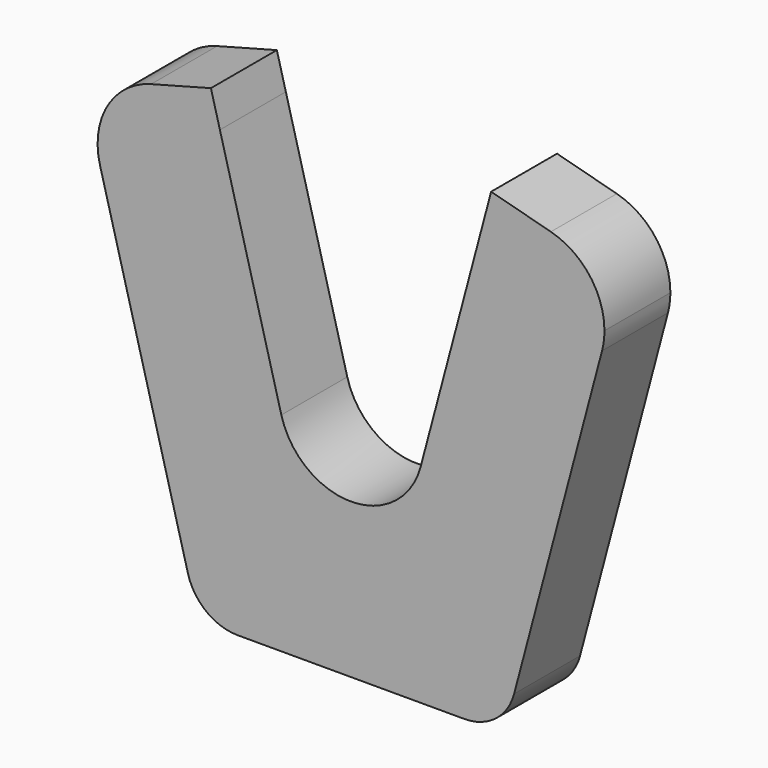
from build123d import *

# Parameters (mm, degrees)
F1_DEPTH = 25.4


with BuildPart() as f1:
    # F0 (on Front) → F1 (new body)
    with BuildSketch(Plane.XZ):
        with BuildLine():
            ThreePointArc((-96.2938510095, 49.8640834202), (-106.1566639379, 55.4102805892), (-117.4718999148, 55.3817029315))
            ThreePointArc((-117.4718999148, 55.3817029315), (-130.9864974324, 45.0518805264), (-133.238473511, 28.1913295056))
            ThreePointArc((-133.238473511, 28.1913295056), (-111.9975569081, 11.6794990469), (-90.4085331471, 27.7335059074))
            Line((-90.4085331471, 27.7335059074), (-96.2938510095, 49.8640834202))
        make_face()
        with BuildLine():
            Line((-99.0630919931, 60.2772681748), (-117.4718999148, 55.3817029315))
            ThreePointArc((-117.4718999148, 55.3817029315), (-106.1566639379, 55.4102805892), (-96.2938510095, 49.8640834202))
            Line((-96.2938510095, 49.8640834202), (-99.0630919931, 60.2772681748))
        make_face()
        with BuildLine():
            ThreePointArc((-90.4085331471, 27.7335059074), (-111.9975569081, 11.6794990469), (-133.238473511, 28.1913295056))
            Line((-133.238473511, 28.1913295056), (-106.1467650121, -73.6816990901))
            ThreePointArc((-106.1467650121, -73.6816990901), (-92.8623116551, -53.860643351), (-74.9299982186, -69.6017705795))
            ThreePointArc((-74.9299982186, -69.6017705795), (-79.5796780672, -80.8270907309), (-90.8049982186, -85.4767705795))
            Line((-90.8049982186, -85.4767705795), (-20.9549982186, -85.4767705795))
            ThreePointArc((-20.9549982186, -85.4767705795), (-32.1803231924, -58.3764516879), (-5.0800017814, -69.6017705795))
            ThreePointArc((-5.0800017814, -69.6017705795), (-5.2138745529, -71.659084016), (-5.6132349879, -73.6816990901))
            Line((-5.6132349879, -73.6816990901), (21.478473511, 28.1913295056))
            ThreePointArc((21.478473511, 28.1913295056), (0.2375569081, 11.6794990469), (-21.3514668529, 27.7335059074))
            Line((-21.3514668529, 27.7335059074), (-34.401526489, -21.3386704944))
            ThreePointArc((-34.401526489, -21.3386704944), (-55.88, -37.8517705795), (-77.358473511, -21.3386704944))
            Line((-77.358473511, -21.3386704944), (-90.4085331471, 27.7335059074))
        make_face()
        with BuildLine():
            ThreePointArc((-74.9299982186, -69.6017705795), (-92.8623116551, -53.860643351), (-106.1467650121, -73.6816990901))
            ThreePointArc((-106.1467650121, -73.6816990901), (-100.4809157434, -82.1871686683), (-90.8049982186, -85.4767705795))
            ThreePointArc((-90.8049982186, -85.4767705795), (-79.5796780672, -80.8270907309), (-74.9299982186, -69.6017705795))
        make_face()
        with BuildLine():
            ThreePointArc((-5.0800017814, -69.6017705795), (-32.1803231924, -58.3764516879), (-20.9549982186, -85.4767705795))
            ThreePointArc((-20.9549982186, -85.4767705795), (-11.2790828443, -82.1871675825), (-5.6132349879, -73.6816990901))
            ThreePointArc((-5.6132349879, -73.6816990901), (-5.2138745529, -71.659084016), (-5.0800017814, -69.6017705795))
        make_face()
        with BuildLine():
            Line((-15.4661489905, 49.8640834202), (-21.3514668529, 27.7335059074))
            ThreePointArc((-21.3514668529, 27.7335059074), (0.2375569081, 11.6794990469), (21.478473511, 28.1913295056))
            ThreePointArc((21.478473511, 28.1913295056), (22.0375781199, 31.0229906094), (22.225, 33.9032294205))
            ThreePointArc((22.225, 33.9032294205), (17.6195573243, 47.4495139552), (5.7118999148, 55.3817029315))
            ThreePointArc((5.7118999148, 55.3817029315), (-5.6033360621, 55.4102805892), (-15.4661489905, 49.8640834202))
        make_face()
        with BuildLine():
            Line((-12.6969080069, 60.2772681748), (-15.4661489905, 49.8640834202))
            ThreePointArc((-15.4661489905, 49.8640834202), (-5.6033360621, 55.4102805892), (5.7118999148, 55.3817029315))
            Line((5.7118999148, 55.3817029315), (-12.6969080069, 60.2772681748))
        make_face()
    extrude(amount=F1_DEPTH)


solid = f1.part
